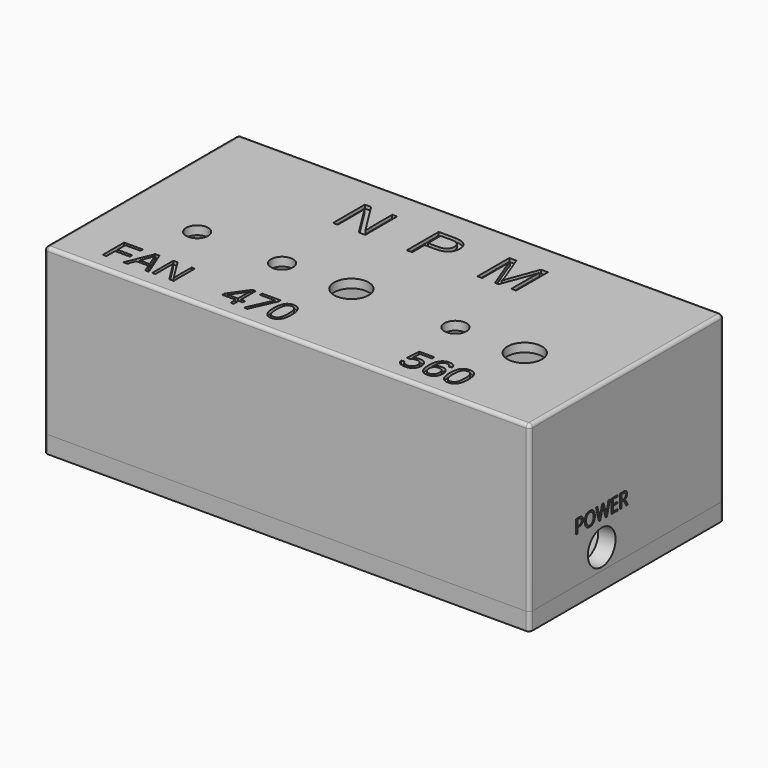
from build123d import *

# Parameters (mm, degrees)
F0_W             = 140
F0_H             = 70
F0_R             = 3.175
F0_R_2           = 5
F1_DEPTH         = 2.5
F2_W             = 140
F2_H             = 70
F2_W_2           = 130
F2_H_2           = 60
F3_DEPTH         = 45
F4_W             = 140
F4_H             = 70
F4_W_2           = 130
F4_H_2           = 60
F5_DEPTH         = 5
F7_D             = 2.4
F7_DEPTH         = 5
F7_CSINK_D       = 4
F7_CSINK_ANGLE   = 90
F7_TIP           = 0.7210327428
F7_2_D           = 2.4
F7_2_DEPTH       = 5
F7_2_CSINK_D     = 4
F7_2_CSINK_ANGLE = 90
F7_2_TIP         = 0.7210327428
F9_D             = 2.9
F9_DEPTH         = 5.2
F9_CBORE_D       = 3.7
F9_CBORE_DEPTH   = 0.2
F9_TIP           = 0.8712478976
F10_R            = 1
F10_2_R          = 1
F13_TEXT_SIZE    = 16.6666666667
F14_DEPTH        = 1
F16_TEXT_SIZE    = 11.1111111111
F17_DEPTH        = 1
F11_R            = 5
F19_DEPTH        = 25
F12_R            = 5
F20_DEPTH        = 25
F21_TEXT_SIZE    = 5.5555555556
F22_DEPTH        = 2
F23_TEXT_SIZE    = 5.5555555556
F24_DEPTH        = 2
F25_R            = 1


# Not quite as in the source:
# - Text() gives the source's letters only with a copy of the font that has no kerning and outlines rounded to 1/6400 em; it was checked with that copy


with BuildPart() as f1:
    # F0 (on Top) → F1 (new body)
    with BuildSketch(Plane.XY):
        with Locations((70, 35)):
            Rectangle(F0_W, F0_H)
        with Locations((22.5, 27)):
            Circle(F0_R, mode=Mode.SUBTRACT)
        with Locations((47, 27)):
            Circle(F0_R, mode=Mode.SUBTRACT)
        with Locations((67, 27)):
            Circle(F0_R_2, mode=Mode.SUBTRACT)
        with Locations((97, 27)):
            Circle(F0_R, mode=Mode.SUBTRACT)
        with Locations((117, 27)):
            Circle(F0_R_2, mode=Mode.SUBTRACT)
    extrude(amount=F1_DEPTH)

    # F2 (on face) → F3 (join)
    with BuildSketch(Plane(origin=(0, 0, 0), x_dir=(1, 0, 0), z_dir=(0, 0, -1))):
        with Locations((70, -35)):
            Rectangle(F2_W, F2_H)
        with Locations((70, -35)):
            Rectangle(F2_W_2, F2_H_2, mode=Mode.SUBTRACT)
    extrude(amount=F3_DEPTH)

    # F7
    with Locations(Plane(origin=(0, 0, -50), x_dir=(1, 0, 0), z_dir=(0, 0, -1))):
        with Locations((2.5, -2.5), (2.5, -67.5), (137.5, -67.5), (137.5, -2.5)):
            CounterSinkHole(F7_D / 2, F7_CSINK_D / 2, depth=F7_DEPTH, counter_sink_angle=F7_CSINK_ANGLE)
            with Locations((0, 0, -(F7_DEPTH + F7_TIP / 2))):  # 118° drill point
                Cone(0, F7_D / 2, F7_TIP, mode=Mode.SUBTRACT)

    # F9
    with Locations(Plane(origin=(0, 0, -45), x_dir=(1, 0, 0), z_dir=(0, 0, -1))):
        with Locations((2.5, -2.5), (2.5, -67.5), (137.5, -67.5), (137.5, -2.5)):
            CounterBoreHole(F9_D / 2, F9_CBORE_D / 2, F9_CBORE_DEPTH, depth=F9_DEPTH)
            with Locations((0, 0, -(F9_DEPTH + F9_TIP / 2))):  # 118° drill point
                Cone(0, F9_D / 2, F9_TIP, mode=Mode.SUBTRACT)

    # F10
    f10_edges = [f1.edges().sort_by_distance(p)[0] for p in [
        (70, 0, 2.5),
        (0, 35, 2.5),
        (70, 70, 2.5),
        (140, 35, 2.5),
        (140, 0, -21.25),
        (0, 0, -21.25),
        (140, 70, -21.25),
        (0, 70, -21.25),
    ]]
    fillet(f10_edges, radius=F10_R)

    # F13 (on face) → F14 (cut)
    with BuildSketch(Plane.XY.offset(2.5)):
        with Locations((42.3268229167, 49.5)):
            Text('N  P  M', F13_TEXT_SIZE, font='Arimo', text_align=(TextAlign.LEFT, TextAlign.BOTTOM))
    extrude(amount=-F14_DEPTH, mode=Mode.SUBTRACT)

    # F15: union 

    # F16 (on face) → F17 (cut)
    with BuildSketch(Plane.XY.offset(2.5)):
        with Locations((12, 5)):
            Text('FAN', F16_TEXT_SIZE, font='Arimo', text_align=(TextAlign.LEFT, TextAlign.BOTTOM))
        with Locations((97.1267361111, 5)):
            Text('560', F16_TEXT_SIZE, font='Arimo', text_align=(TextAlign.LEFT, TextAlign.BOTTOM))
        with Locations((45.9010416667, 4.7221066505)):
            Text('470', F16_TEXT_SIZE, font='Open Sans', text_align=(TextAlign.LEFT, TextAlign.BOTTOM))
    extrude(amount=-F17_DEPTH, mode=Mode.SUBTRACT)

    # F11 (on face) → F19 (cut)
    with BuildSketch(Plane(origin=(0, 0, 0), x_dir=(0, -1, 0), z_dir=(-1, 0, 0))):
        with Locations((-20, -39)):
            Circle(F11_R)
        with Locations((-35, -39)):
            Circle(F11_R)
        with Locations((-50, -39)):
            Circle(F11_R)
    extrude(amount=-F19_DEPTH, mode=Mode.SUBTRACT)

    # F12 (on face) → F20 (cut)
    with BuildSketch(Plane.YZ.offset(140)):
        with Locations((26, -39)):
            Circle(F12_R)
    extrude(amount=-F20_DEPTH, mode=Mode.SUBTRACT)

    # F21 (on face) → F22 (cut)
    with BuildSketch(Plane(origin=(0, 0, 0), x_dir=(0, -1, 0), z_dir=(-1, 0, 0))):
        with Locations((-54.5, -32)):
            Text('FAN   470    560', F21_TEXT_SIZE, font='Open Sans', text_align=(TextAlign.LEFT, TextAlign.BOTTOM))
    extrude(amount=-F22_DEPTH, mode=Mode.SUBTRACT)

    # F23 (on face) → F24 (cut)
    with BuildSketch(Plane.YZ.offset(140)):
        with Locations((16.1983506944, -32)):
            Text('POWER', F23_TEXT_SIZE, font='Open Sans', text_align=(TextAlign.LEFT, TextAlign.BOTTOM))
    extrude(amount=-F24_DEPTH, mode=Mode.SUBTRACT)

    # F25
    f25_edges = [f1.edges().sort_by_distance(p)[0] for p in [
        (5, 5, -22.5),
        (135, 5, -22.5),
        (135, 65, -22.5),
        (5, 65, -22.5),
    ]]
    fillet(f25_edges, radius=F25_R)


with BuildPart() as f5:
    # F4 (on face) → F5 (new body)
    with BuildSketch(Plane(origin=(0, 0, -45), x_dir=(1, 0, 0), z_dir=(0, 0, -1))):
        with Locations((70, -35)):
            Rectangle(F4_W, F4_H)
        with Locations((70, -35)):
            Rectangle(F4_W_2, F4_H_2, mode=Mode.SUBTRACT)
        with Locations((70, -35)):
            Rectangle(F4_W_2, F4_H_2)
    extrude(amount=F5_DEPTH)

    # F7#2
    with Locations(Plane(origin=(0, 0, -50), x_dir=(1, 0, 0), z_dir=(0, 0, -1))):
        with Locations((2.5, -2.5), (2.5, -67.5), (137.5, -67.5), (137.5, -2.5)):
            CounterSinkHole(F7_2_D / 2, F7_2_CSINK_D / 2, depth=F7_2_DEPTH, counter_sink_angle=F7_2_CSINK_ANGLE)
            with Locations((0, 0, -(F7_2_DEPTH + F7_2_TIP / 2))):  # 118° drill point
                Cone(0, F7_2_D / 2, F7_2_TIP, mode=Mode.SUBTRACT)

    # F10#2
    f10_2_edges = [f5.edges().sort_by_distance(p)[0] for p in [
        (0, 70, -47.5),
        (0, 0, -47.5),
        (140, 70, -47.5),
        (140, 0, -47.5),
    ]]
    fillet(f10_2_edges, radius=F10_2_R)


solid = Compound([f1.part, f5.part])
